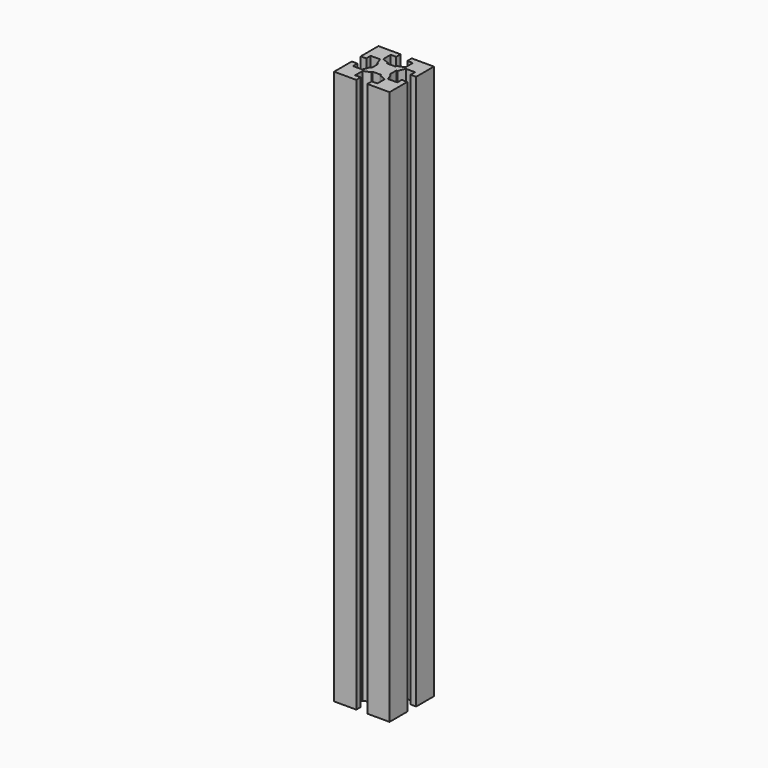
from build123d import *

# Parameters (mm, degrees)
F1_DEPTH = 75


# Not quite as in the source:
# - ends of sketch curves that miss each other by under 0.0002 mm in the source are joined


with BuildPart() as f1:
    # F0 (on Top) → F1 (new body, symmetric)
    with BuildSketch(Plane.XY):
        Polygon((7.5, 1.5), (7.5, 7.5), (1.5, 7.5), (1.5, 6), (3, 6), (3, 3.5), (1.1461396934, 2.7563427575), (1.1461396934, 2.42764467), (-1.1461396934, 2.42764467), (-1.1461396934, 2.7563427575), (-3, 3.5), (-3, 6), (-1.5, 6), (-1.5, 7.5), (-7.5, 7.5), (-7.5, 1.5), (-6, 1.5), (-6, 3), (-3.5, 3), (-2.7563427575, 1.1461396934), (-2.42764467, 1.1461396934), (-2.42764467, -1.1461396934), (-2.7563427575, -1.1461396934), (-3.5, -3), (-6, -3), (-6, -1.5), (-7.5, -1.5), (-7.5, -7.5), (-1.5, -7.5), (-1.5, -6), (-3, -6), (-3, -3.5), (-1.1461396934, -2.7563427575), (-1.1461396934, -2.42764467), (1.1461396934, -2.42764467), (1.1461396934, -2.7563427575), (3, -3.5), (3, -6), (1.5, -6), (1.5, -7.5), (7.5, -7.5), (7.5, -1.5), (6, -1.5), (6, -3), (3.5, -3), (2.7563427575, -1.1461396934), (2.42764467, -1.1461396934), (2.42764467, 1.1461396934), (2.7563427575, 1.1461396934), (3.5, 3), (6, 3), (6, 1.5), align=None)
    extrude(amount=F1_DEPTH, both=True)


solid = f1.part
